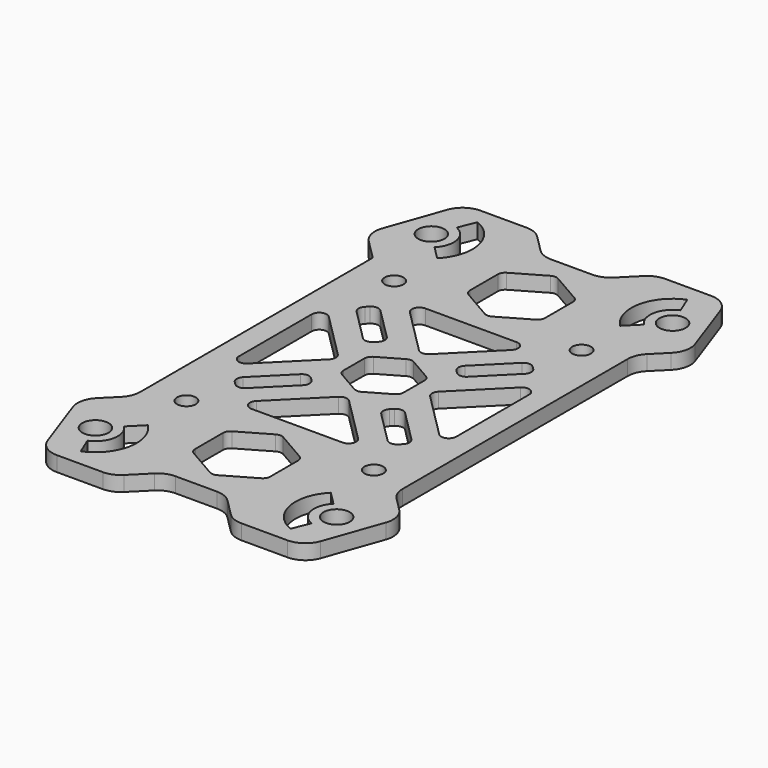
from build123d import *

# Parameters (mm, degrees)
F0_R     = 1.75
F0_R_2   = 1.25
F1_DEPTH = 2
F2_R     = 3
F3_R     = 1


# Not quite as in the source:
# - a feature names something its author has since deleted; it is built from what else it names


with BuildPart() as f1:
    # F0 (on Top) → F1 (new body)
    with BuildSketch(Plane.XY):
        Polygon((-21.5, 24), (-17.5, 20), (-17.5, -20), (-21.5, -24), (-17.5, -35.313708499), (-8, -35.313708499), (-4, -31.313708499), (4, -31.313708499), (8, -35.313708499), (17.5, -35.313708499), (21.5, -24), (17.5, -20), (17.5, 20), (21.5, 24), (17.5, 35.313708499), (8, 35.313708499), (4, 31.313708499), (-4, 31.313708499), (-8, 35.313708499), (-17.5, 35.313708499), align=None)
        with Locations((-16.0857864376, -28)):
            Circle(F0_R, mode=Mode.SUBTRACT)
        with BuildLine():
            Line((-13.9644660941, -25.8786796564), (-12.1966991411, -24.1109127035))
            ThreePointArc((-12.1966991411, -24.1109127035), (-10.6914673954, -29.0729967711), (-13.9810275596, -33.0813374288))
            Line((-13.9810275596, -33.0813374288), (-14.9377361405, -30.7716385975))
            ThreePointArc((-14.9377361405, -30.7716385975), (-13.1434305964, -28.585270966), (-13.9644660941, -25.8786796564))
        make_face(mode=Mode.SUBTRACT)
        with Locations((-12.5, -17.313708499)):
            Circle(F0_R_2, mode=Mode.SUBTRACT)
        Polygon((-8.4895923599, -14.5), (0, -6.0104076401), (8.4895923599, -14.5), align=None, mode=Mode.SUBTRACT)
        Polygon((-11.9246212025, -10.1568542495), (-10.8838834765, -9.1161165235), (-6.267766953, -4.5), (-4.5, -6.267766953), (-9.1161165302, -10.8838834832), (-10.1568542495, -11.9246212025), align=None, mode=Mode.SUBTRACT)
        Polygon((0, -28.6803569414), (-5, -25.7936055954), (-5, -20.0201029035), (0, -17.1333515576), (5, -20.0201029035), (5, -25.7936055954), align=None, mode=Mode.SUBTRACT)
        with BuildLine():
            ThreePointArc((13.9644660941, -25.8786796564), (13.1434305964, -28.585270966), (14.9377361405, -30.7716385975))
            Line((14.9377361405, -30.7716385975), (13.9810275596, -33.0813374288))
            ThreePointArc((13.9810275596, -33.0813374288), (10.6914673954, -29.0729967711), (12.1966991411, -24.1109127035))
            Line((12.1966991411, -24.1109127035), (13.9644660941, -25.8786796564))
        make_face(mode=Mode.SUBTRACT)
        with Locations((16.0857864376, -28)):
            Circle(F0_R, mode=Mode.SUBTRACT)
        Polygon((6.267766953, -4.5), (10.8838834914, -9.1161165384), (11.9246212025, -10.1568542495), (10.1568542495, -11.9246212025), (9.1161165343, -10.8838834873), (4.5, -6.267766953), align=None, mode=Mode.SUBTRACT)
        with Locations((12.5, -17.313708499)):
            Circle(F0_R_2, mode=Mode.SUBTRACT)
        with Locations((-12.5, 17.313708499)):
            Circle(F0_R_2, mode=Mode.SUBTRACT)
        Polygon((-14.5, 8.4895923599), (-6.0104076401, 0), (-14.5, -8.4895923599), align=None, mode=Mode.SUBTRACT)
        Polygon((-10.1568542495, 11.9246212025), (-9.1161165117, 10.8838834647), (-4.5, 6.267766953), (-6.267766953, 4.5), (-10.8838834765, 9.1161165235), (-11.9246212025, 10.1568542495), align=None, mode=Mode.SUBTRACT)
        with Locations((-16.0857864376, 28)):
            Circle(F0_R, mode=Mode.SUBTRACT)
        with BuildLine():
            Line((-12.1966991411, 24.1109127035), (-13.9644660941, 25.8786796564))
            ThreePointArc((-13.9644660941, 25.8786796564), (-13.1434305964, 28.585270966), (-14.9377361405, 30.7716385975))
            Line((-14.9377361405, 30.7716385975), (-13.9810275596, 33.0813374288))
            ThreePointArc((-13.9810275596, 33.0813374288), (-10.6914673954, 29.0729967711), (-12.1966991411, 24.1109127035))
        make_face(mode=Mode.SUBTRACT)
        Polygon((0, -4.6188021535), (-4, -2.3094010768), (-4, 2.3094010768), (0, 4.6188021535), (4, 2.3094010768), (4, -2.3094010768), align=None, mode=Mode.SUBTRACT)
        Polygon((14.5, -8.4895923599), (6.0104076401, 0), (14.5, 8.4895923599), align=None, mode=Mode.SUBTRACT)
        Polygon((4.5, 6.267766953), (9.1161165235, 10.8838834765), (10.1568542495, 11.9246212025), (11.9246212025, 10.1568542495), (10.8838834765, 9.1161165235), (6.267766953, 4.5), align=None, mode=Mode.SUBTRACT)
        Polygon((0, 6.0104076401), (-8.4895923599, 14.5), (8.4895923599, 14.5), align=None, mode=Mode.SUBTRACT)
        with Locations((12.5, 17.313708499)):
            Circle(F0_R_2, mode=Mode.SUBTRACT)
        Polygon((0, 17.1333515576), (-5, 20.0201029035), (-5, 25.7936055954), (0, 28.6803569414), (5, 25.7936055954), (5, 20.0201029035), align=None, mode=Mode.SUBTRACT)
        with BuildLine():
            Line((13.9644660941, 25.8786796564), (12.1966991411, 24.1109127035))
            ThreePointArc((12.1966991411, 24.1109127035), (10.6914673954, 29.0729967711), (13.9810275596, 33.0813374288))
            Line((13.9810275596, 33.0813374288), (14.9377361405, 30.7716385975))
            ThreePointArc((14.9377361405, 30.7716385975), (13.1434305964, 28.585270966), (13.9644660941, 25.8786796564))
        make_face(mode=Mode.SUBTRACT)
        with Locations((16.0857864376, 28)):
            Circle(F0_R, mode=Mode.SUBTRACT)
    extrude(amount=F1_DEPTH)

    # F2
    f2_edges = [f1.edges().sort_by_distance(p)[0] for p in [
        (-21.5, -24, 1),
        (-17.5, -20, 1),
        (-17.5, -35.313708, 1),
        (17.5, -35.313708, 1),
        (21.5, -24, 1),
        (17.5, -20, 1),
        (17.5, 20, 1),
        (21.5, 24, 1),
        (17.5, 35.313708, 1),
        (-17.5, 35.313708, 1),
        (-21.5, 24, 1),
        (-8, -35.313708, 1),
        (-4, -31.313708, 1),
        (4, -31.313708, 1),
        (8, -35.313708, 1),
        (-8, 35.313708, 1),
        (-4, 31.313708, 1),
        (4, 31.313708, 1),
        (8, 35.313708, 1),
    ]]
    fillet(f2_edges, radius=F2_R)

    # F3
    f3_edges = [f1.edges().sort_by_distance(p)[0] for p in [
        (-10.156854, 11.924621, 1),
        (-11.924621, 10.156854, 1),
        (-4.5, 6.267767, 1),
        (-6.267767, 4.5, 1),
        (10.156854, 11.924621, 1),
        (11.924621, 10.156854, 1),
        (6.267767, 4.5, 1),
        (4.5, 6.267767, 1),
        (-11.924621, -10.156854, 1),
        (4.5, -6.267767, 1),
        (-4.5, -6.267767, 1),
        (11.924621, -10.156854, 1),
        (10.156854, -11.924621, 1),
        (-10.156854, -11.924621, 1),
        (-6.267767, -4.5, 1),
        (6.267767, -4.5, 1),
        (5, 20.020103, 1),
        (5, 25.793606, 1),
        (0, 28.680357, 1),
        (-5, 25.793606, 1),
        (-5, 20.020103, 1),
        (0, 17.133352, 1),
        (8.489592, -14.5, 1),
        (-8.489592, -14.5, 1),
        (0, -6.010408, 1),
        (0, 6.010408, 1),
        (8.489592, 14.5, 1),
        (-8.489592, 14.5, 1),
        (-6.010408, 0, 1),
        (-14.5, 8.489592, 1),
        (-14.5, -8.489592, 1),
        (14.5, 8.489592, 1),
        (6.010408, 0, 1),
        (14.5, -8.489592, 1),
        (-5, -20.020103, 1),
        (0, -17.133352, 1),
        (5, -20.020103, 1),
        (5, -25.793606, 1),
        (0, -28.680357, 1),
        (-5, -25.793606, 1),
        (4, 2.309401, 1),
        (4, -2.309401, 1),
        (0, -4.618802, 1),
        (-4, -2.309401, 1),
        (-4, 2.309401, 1),
        (0, 4.618802, 1),
    ]]
    fillet(f3_edges, radius=F3_R)


solid = f1.part
